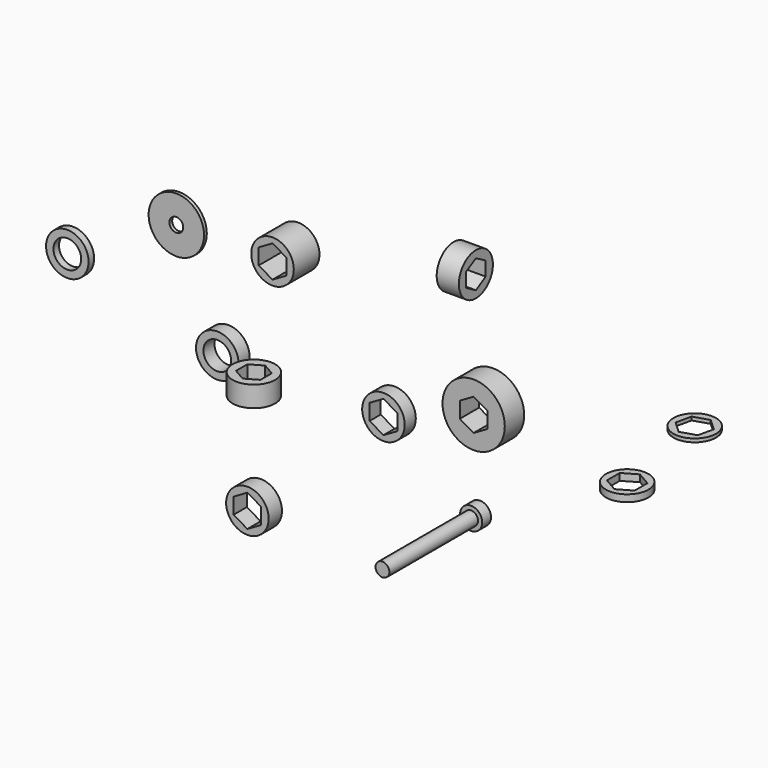
from build123d import *

# Parameters (mm, degrees)
F0_R      = 9.7536
F1_DEPTH  = 6.35
F2_R      = 9.7536
F3_DEPTH  = 9.525
F4_R      = 9.7536
F5_DEPTH  = 10.16
F6_R      = 9.7536
F7_DEPTH  = 3.175
F8_R      = 9.7536
F8_R_2    = 6.35
F9_DEPTH  = 6.35
F10_R     = 9.7536
F11_DEPTH = 1.5875
F12_R     = 9.7536
F12_R_2   = 6.35
F13_DEPTH = 3.175
F14_R     = 14.2875
F15_DEPTH = 11.1125
F16_R     = 9.7536
F17_DEPTH = 14.71168
F18_R     = 12.7
F18_R_2   = 3.175
F20_DEPTH = 1.5875
F19_R     = 9.7536
F21_DEPTH = 7.62
F22_R     = 5.08
F23_DEPTH = 5.08
F24_R     = 3.175
F25_DEPTH = 50.8


# Not quite as in the source:
# - a length typed as a fraction of an inch, garbled in the dataset ("3 / 203.2 mm" for 3/8 in), is restored


with BuildPart() as f1:
    # F0 (on Front) → F1 (new body)
    with BuildSketch(Plane.XZ):
        Circle(F0_R)
        Polygon((0, 7.3323484187), (6.35, 3.6661742094), (6.35, -3.6661742094), (0, -7.3323484187), (-6.35, -3.6661742094), (-6.35, 3.6661742094), align=None, mode=Mode.SUBTRACT)
    extrude(amount=F1_DEPTH)


with BuildPart() as f3:
    # F2 (on Top) → F3 (new body)
    with BuildSketch(Plane.XY):
        with Locations((-46.5451255441, -22.4268511866)):
            Circle(F2_R)
        Polygon((-46.5451255441, -15.9498511866), (-40.9358790038, -19.1883511866), (-40.9358790038, -25.6653511866), (-46.5451255441, -28.9038511866), (-52.1543720844, -25.6653511866), (-52.1543720844, -19.1883511866), align=None, mode=Mode.SUBTRACT)
    extrude(amount=F3_DEPTH)


with BuildPart() as f5:
    # F4 (on Right) → F5 (new body)
    with BuildSketch(Plane.YZ):
        with Locations((33.922277391, 44.5486380722)):
            Circle(F4_R)
        Polygon((33.922277391, 51.0256380722), (39.5315239313, 47.7871380722), (39.5315239313, 41.3101380722), (33.922277391, 38.0716380722), (28.3130308506, 41.3101380722), (28.3130308506, 47.7871380722), align=None, mode=Mode.SUBTRACT)
    extrude(amount=F5_DEPTH)


with BuildPart() as f7:
    # F6 (on Top) → F7 (new body)
    with BuildSketch(Plane.XY):
        with Locations((103.3476446891, 4.1662805695)):
            Circle(F6_R)
        Polygon((103.3476446891, 11.4986289883), (109.6976446891, 7.8324547789), (109.6976446891, 0.5001063602), (103.3476446891, -3.1660678492), (96.9976446891, 0.5001063602), (96.9976446891, 7.8324547789), align=None, mode=Mode.SUBTRACT)
    extrude(amount=F7_DEPTH)


with BuildPart() as f9:
    # F8 (on Front) → F9 (new body)
    with BuildSketch(Plane.XZ):
        with Locations((-76.2, 0)):
            Circle(F8_R)
        with Locations((-76.2, 0)):
            Circle(F8_R_2, mode=Mode.SUBTRACT)
    extrude(amount=F9_DEPTH)


with BuildPart() as f11:
    # F10 (on Top) → F11 (new body)
    with BuildSketch(Plane.XY):
        with Locations((93.2527035475, 55.487845093)):
            Circle(F10_R)
        Polygon((94.8433153394, 62.6455882751), (100.2467968729, 57.6892064647), (98.656185081, 50.5314632826), (91.6620917556, 48.3301019109), (86.2586102221, 53.2864837213), (87.849222014, 60.4442269034), align=None, mode=Mode.SUBTRACT)
    extrude(amount=F11_DEPTH)


with BuildPart() as f13:
    # F12 (on Front) → F13 (new body)
    with BuildSketch(Plane.XZ):
        with Locations((-147.4970877171, 16.5493860841)):
            Circle(F12_R)
        with Locations((-147.4970877171, 16.5493860841)):
            Circle(F12_R_2, mode=Mode.SUBTRACT)
    extrude(amount=F13_DEPTH)


with BuildPart() as f15:
    # F14 (on Front) → F15 (new body)
    with BuildSketch(Plane.XZ):
        with Locations((45.1609123334, 17.4948293716)):
            Circle(F14_R)
        Polygon((45.1609123334, 24.8271777903), (51.5109123334, 21.1610035809), (51.5109123334, 13.8286551622), (45.1609123334, 10.1624809529), (38.8109123334, 13.8286551622), (38.8109123334, 21.1610035809), align=None, mode=Mode.SUBTRACT)
    extrude(amount=F15_DEPTH)


with BuildPart() as f17:
    # F16 (on Front) → F17 (new body)
    with BuildSketch(Plane.XZ):
        with Locations((-44.1768842667, 51.7929382622)):
            Circle(F16_R)
        Polygon((-44.1768842667, 59.1252866809), (-37.8268842667, 55.4591124716), (-37.8268842667, 48.1267640529), (-44.1768842667, 44.4605898435), (-50.5268842667, 48.1267640529), (-50.5268842667, 55.4591124716), align=None, mode=Mode.SUBTRACT)
    extrude(amount=F17_DEPTH)


with BuildPart() as f20:
    # F18 (on Front) → F20 (new body)
    with BuildSketch(Plane.XZ):
        with Locations((-98.7787470222, 43.4638410807)):
            Circle(F18_R)
        with Locations((-98.7787470222, 43.4638410807)):
            Circle(F18_R_2, mode=Mode.SUBTRACT)
    extrude(amount=F20_DEPTH)


with BuildPart() as f21:
    # F19 (on Front) → F21 (new body)
    with BuildSketch(Plane.XZ):
        with Locations((-61.3744067824, -57.3208441976)):
            Circle(F19_R)
        Polygon((-61.3744067824, -49.9884957789), (-55.0244067824, -53.6546699883), (-55.0244067824, -60.987018407), (-61.3744067824, -64.6531926163), (-67.7244067824, -60.987018407), (-67.7244067824, -53.6546699883), align=None, mode=Mode.SUBTRACT)
    extrude(amount=F21_DEPTH)


with BuildPart() as f23:
    # F22 (on Front) → F23 (new body)
    with BuildSketch(Plane.XZ):
        with Locations((39.1776077449, -28.6891143769)):
            Circle(F22_R)
    extrude(amount=F23_DEPTH)

    # F24 (on face) → F25 (join)
    with BuildSketch(Plane.XZ.offset(5.08)):
        with Locations((39.1776077449, -28.6891143769)):
            Circle(F24_R)
    extrude(amount=F25_DEPTH)


solid = Compound([f1.part, f3.part, f5.part, f7.part, f9.part, f11.part, f13.part, f15.part, f17.part, f20.part, f21.part, f23.part])
